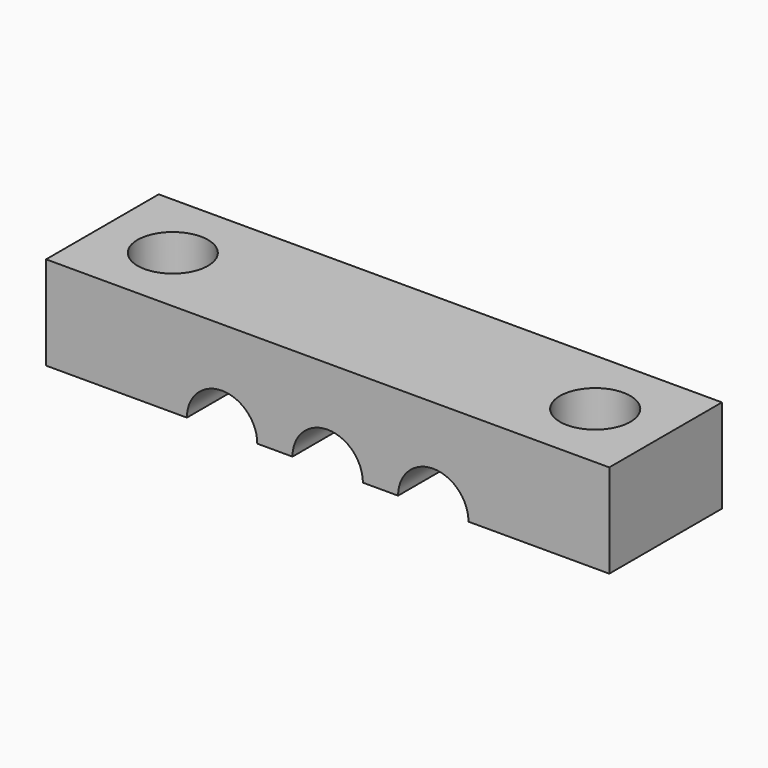
from build123d import *

# Parameters (mm, degrees)
F2_DEPTH = 12.7
F4_D     = 6.35


# Not quite as in the source:
# - a variable given as a bare number and used for a length is read in inches; the dataset says mm whatever the document's units were


with BuildPart() as f2:
    # F1 (on Front) → F2 (new body)
    with BuildSketch(Plane.XZ):
        with BuildLine():
            Line((-25.4, 8.4416426996), (-25.4, 0))
            Line((-25.4, 0), (-12.7, 0))
            ThreePointArc((-12.7, 0), (-9.525, 3.175), (-6.35, 0))
            Line((-6.35, 0), (-3.175, 0))
            ThreePointArc((-3.175, 0), (0, 3.175), (3.175, 0))
            Line((3.175, 0), (6.35, 0))
            ThreePointArc((6.35, 0), (9.525, 3.175), (12.7, 0))
            Line((12.7, 0), (25.4, 0))
            Line((25.4, 0), (25.4, 8.4416426996))
            Line((25.4, 8.4416426996), (-25.4, 8.4416426996))
        make_face()
    extrude(amount=F2_DEPTH)

    # F4 (through all)
    with Locations(Plane.XY.offset(8.4416426996)):
        with Locations((-19.05, -6.35), (19.05, -6.35)):
            Hole(F4_D / 2)


solid = f2.part
